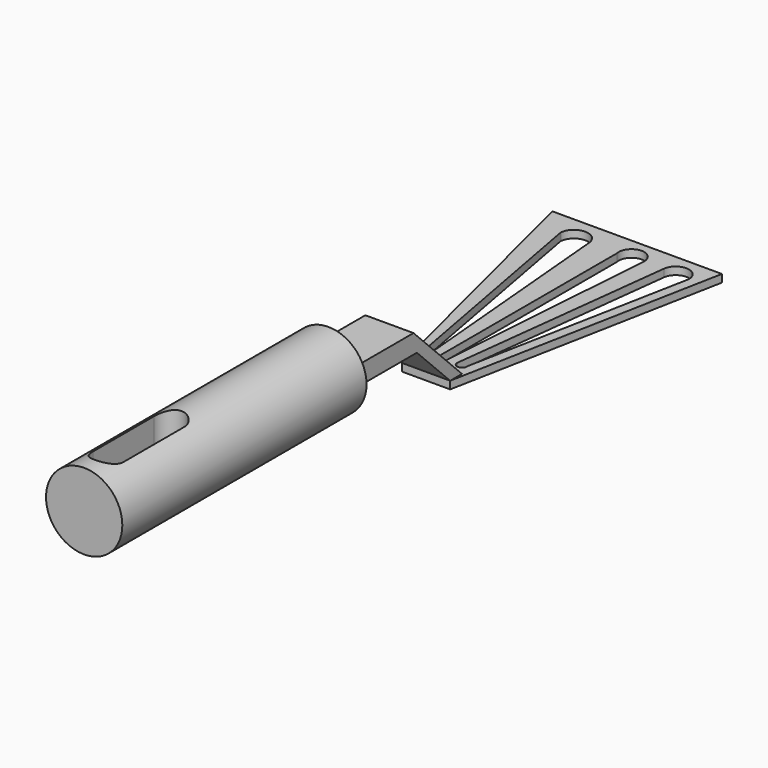
from build123d import *

# Parameters (mm, degrees)
F0_R        = 12.7
F1_DEPTH    = 101.6
F3_DEPTH    = 12.7
F4_W        = 16.0404779017
F4_H        = 6.3281008042
F5_DEPTH    = 25.4
F6_W        = 16.0404779017
F6_H        = 20.1715745497
F7_DEPTH    = 25.4
F8_T1_DEPTH = 146.6819736904
F9_T4_DEPTH = 94.4253753749
F11_DEPTH   = 2.54
F13_DEPTH   = 2.54


# Not quite as in the source:
# - a fillet or chamfer that OpenCascade refuses, or shapes differently, is made with other operations: its cross-section is extruded or revolved along the edge and cut away or added


with BuildPart() as f1:
    # F0 (on Front) → F1 (new body)
    with BuildSketch(Plane.XZ):
        Circle(F0_R)
    extrude(amount=F1_DEPTH)

    # F2 (on Top) → F3 (cut, symmetric)
    with BuildSketch(Plane.XY):
        with BuildLine():
            Line((-5.3473415828, -65.8879665646), (-5.3473415828, -91.3225393835))
            ThreePointArc((-5.3473415828, -91.3225393835), (-0.2501727202, -96.3679371527), (4.8125407702, -91.2879665646))
            Line((4.8125407702, -91.2879665646), (4.8125407702, -65.8879665646))
            ThreePointArc((4.8125407702, -65.8879665646), (-0.2674004063, -60.8324133101), (-5.3473415828, -65.8879665646))
        make_face()
    extrude(amount=F3_DEPTH, both=True, mode=Mode.SUBTRACT)

    # F4 (on face) → F5 (join)
    with BuildSketch(Plane(origin=(0, 0, 0), x_dir=(-1, 0, 0), z_dir=(0, 1, 0))):
        Rectangle(F4_W, F4_H)
    extrude(amount=F5_DEPTH)

    # F6 (on face) → F7 (join)
    with BuildSketch(Plane(origin=(0, 25.4, 0), x_dir=(-1, 0, 0), z_dir=(0, 1, 0))):
        with Locations((0, -6.9217368728)):
            Rectangle(F6_W, F6_H)
    extrude(amount=F7_DEPTH)

    # F8: chamfer of 25.4 on 1 edges, made by hand

    # F8_s2 → F8_t1 (cut)
    with BuildSketch(Plane.YZ.offset(-73.3409868452)):
        Polygon((50.8, -22.2359495979), (25.4, 3.1640504021), (50.8, 3.1640504021), align=None)
    extrude(amount=F8_T1_DEPTH, mode=Mode.SUBTRACT)

    # F9: chamfer of 15.24 on 1 edges, made by hand


with BuildPart() as f9_tool2:
    # F9_s3 → F9_t4 (new body)
    with BuildSketch(Plane.YZ.offset(47.2126876874)):
        Polygon((40.64, -17.0075241476), (25.4, -1.7675241476), (25.4, -17.0075241476), align=None)
    extrude(amount=-F9_T4_DEPTH)

    split(bisect_by=Plane.XY.offset(-3.1640504021), keep=Keep.BOTTOM)


with BuildPart() as f1_1:
    add(f1.part)

    # F9_t1: cut F9_tool2
    add(f9_tool2.part, mode=Mode.SUBTRACT)


with BuildPart() as f11:
    # F10 (on face) → F11 (new body)
    with BuildSketch(Plane(origin=(0, 0, -17.0075241476), x_dir=(1, 0, 0), z_dir=(0, 0, -1))):
        Polygon((25.6205989037, -131.7045986652), (8.0202389508, -40.64), (-8.0202389508, -40.64), (-30.8284154249, -131.7045986652), align=None)
    extrude(amount=F11_DEPTH)

    # F12 (on face) → F13 (cut)
    with BuildSketch(Plane.XY.offset(-17.0075241476)):
        with BuildLine():
            ThreePointArc((-2.9510988388, 49.8066730797), (-1.4755494194, 47.3481245776), (0, 49.8066730797))
            Line((0, 49.8066730797), (5.4011049135, 124.3297383189))
            ThreePointArc((5.4011049135, 124.3297383189), (0.9191672956, 128.8501607928), (-2.9510988388, 123.7961500883))
            Line((-2.9510988388, 123.7961500883), (-2.9510988388, 49.8066730797))
        make_face()
        with BuildLine():
            ThreePointArc((-8.0202389508, 49.8066730797), (-6.8753334051, 48.5558313222), (-5.7304278594, 49.8066730797))
            Line((-5.7304278594, 49.8066730797), (-12.2866457498, 123.7961500883))
            ThreePointArc((-12.2866457498, 123.7961500883), (-16.9887549329, 128.1000285349), (-21.690864116, 123.7961500883))
            Line((-21.690864116, 123.7961500883), (-8.0202389508, 49.8066730797))
        make_face()
        with BuildLine():
            Line((6.4293653704, 49.9283634126), (20.7443441266, 123.9943369966))
            ThreePointArc((20.7443441266, 123.9943369966), (16.6519501735, 128.448902691), (11.9976941496, 124.5851293206))
            Line((11.9976941496, 124.5851293206), (3.1607365236, 49.8066730797))
            ThreePointArc((3.1607365236, 49.8066730797), (4.8661303133, 47.9583109849), (6.4293653704, 49.9283634126))
        make_face()
    extrude(amount=-F13_DEPTH, mode=Mode.SUBTRACT)


solid = Compound([f1_1.part, f11.part])
